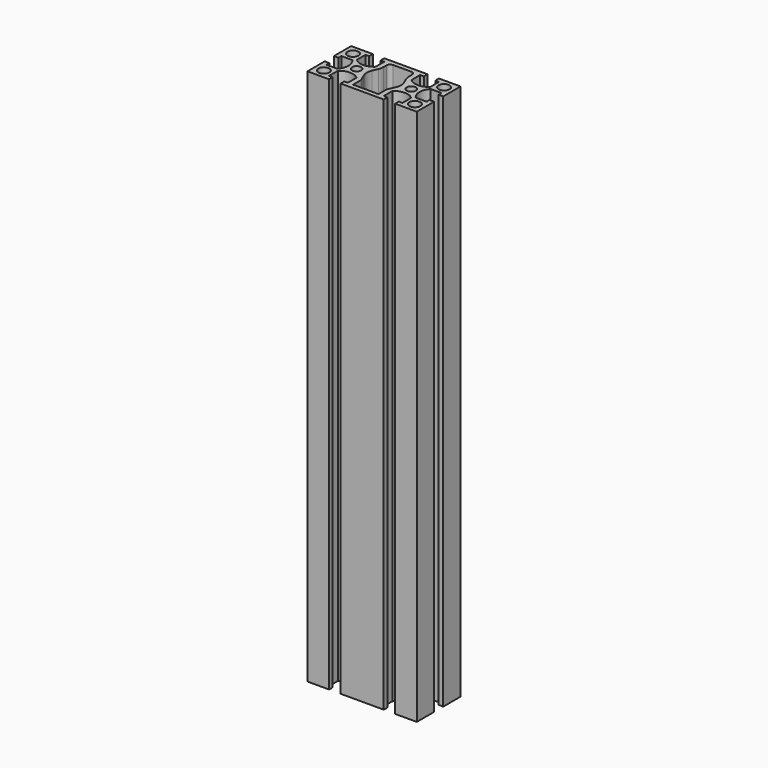
from build123d import *

# Parameters (mm, degrees)
F0_R     = 3
F0_R_2   = 2.5
F1_DEPTH = 295
F2_R     = 2
F3_R     = 7


# Not quite as in the source:
# - a feature names something its author has since deleted; it is built from what else it names


with BuildPart() as f1:
    # F0 (on Top) → F1 (new body)
    with BuildSketch(Plane.XY):
        with BuildLine():
            Line((18.15, -15), (30, -15))
            Line((30, -15), (30, -3.15))
            Line((30, -3.15), (27.5, -3.15))
            Line((27.5, -3.15), (27.5, -5.15))
            Line((27.5, -5.15), (21.5477069044, -5.15))
            ThreePointArc((21.5477069044, -5.15), (19.5, 0), (21.5477069044, 5.15))
            Line((21.5477069044, 5.15), (27.5, 5.15))
            Line((27.5, 5.15), (27.5, 3.15))
            Line((27.5, 3.15), (30, 3.15))
            Line((30, 3.15), (30, 15))
            Line((30, 15), (18.15, 15))
            Line((18.15, 15), (18.15, 12.5))
            Line((18.15, 12.5), (20.15, 12.5))
            Line((20.15, 12.5), (20.15, 6.5477069044))
            ThreePointArc((20.15, 6.5477069044), (15, 4.5), (9.85, 6.5477069044))
            Line((9.85, 6.5477069044), (9.85, 12.5))
            Line((9.85, 12.5), (11.85, 12.5))
            Line((11.85, 12.5), (11.85, 15))
            Line((11.85, 15), (-11.85, 15))
            Line((-11.85, 15), (-11.85, 12.5))
            Line((-11.85, 12.5), (-9.85, 12.5))
            Line((-9.85, 12.5), (-9.85, 6.5477069044))
            ThreePointArc((-9.85, 6.5477069044), (-15, 4.5), (-20.15, 6.5477069044))
            Line((-20.15, 6.5477069044), (-20.15, 12.5))
            Line((-20.15, 12.5), (-18.15, 12.5))
            Line((-18.15, 12.5), (-18.15, 15))
            Line((-18.15, 15), (-30, 15))
            Line((-30, 15), (-30, 3.15))
            Line((-30, 3.15), (-27.5, 3.15))
            Line((-27.5, 3.15), (-27.5, 5.15))
            Line((-27.5, 5.15), (-21.5477069044, 5.15))
            ThreePointArc((-21.5477069044, 5.15), (-19.5, 0), (-21.5477069044, -5.15))
            Line((-21.5477069044, -5.15), (-27.5, -5.15))
            Line((-27.5, -5.15), (-27.5, -3.15))
            Line((-27.5, -3.15), (-30, -3.15))
            Line((-30, -3.15), (-30, -15))
            Line((-30, -15), (-18.15, -15))
            Line((-18.15, -15), (-18.15, -12.5))
            Line((-18.15, -12.5), (-20.15, -12.5))
            Line((-20.15, -12.5), (-20.15, -6.5477069044))
            ThreePointArc((-20.15, -6.5477069044), (-15, -4.5), (-9.85, -6.5477069044))
            Line((-9.85, -6.5477069044), (-9.85, -12.5))
            Line((-9.85, -12.5), (-11.85, -12.5))
            Line((-11.85, -12.5), (-11.85, -15))
            Line((-11.85, -15), (11.85, -15))
            Line((11.85, -15), (11.85, -12.5))
            Line((11.85, -12.5), (9.85, -12.5))
            Line((9.85, -12.5), (9.85, -6.5477069044))
            ThreePointArc((9.85, -6.5477069044), (15, -4.5), (20.15, -6.5477069044))
            Line((20.15, -6.5477069044), (20.15, -12.5))
            Line((20.15, -12.5), (18.15, -12.5))
            Line((18.15, -12.5), (18.15, -15))
        make_face()
        with Locations((-25, -10)):
            Circle(F0_R, mode=Mode.SUBTRACT)
        with Locations((25, -10)):
            Circle(F0_R, mode=Mode.SUBTRACT)
        with Locations((-15, 0)):
            Circle(F0_R_2, mode=Mode.SUBTRACT)
        with Locations((-25, 10)):
            Circle(F0_R, mode=Mode.SUBTRACT)
        Polygon((-7, 7), (-7, 12.5), (0, 12.5), (7, 12.5), (7, 7), (10, 0), (7, -7), (7, -12.5), (0, -12.5), (-7, -12.5), (-7, -7), (-10, 0), align=None, mode=Mode.SUBTRACT)
        with Locations((15, 0)):
            Circle(F0_R_2, mode=Mode.SUBTRACT)
        with Locations((25, 10)):
            Circle(F0_R, mode=Mode.SUBTRACT)
    extrude(amount=F1_DEPTH)

    # F2
    f2_edges = [f1.edges().sort_by_distance(p)[0] for p in [
        (-7, 12.5, 147.5),
        (7, 12.5, 147.5),
    ]]
    fillet(f2_edges, radius=F2_R)

    # F3
    f3_edges = [f1.edges().sort_by_distance(p)[0] for p in [
        (-7, 7, 147.5),
        (-10, 0, 147.5),
        (7, 7, 147.5),
        (10, 0, 147.5),
    ]]
    fillet(f3_edges, radius=F3_R)


solid = f1.part
